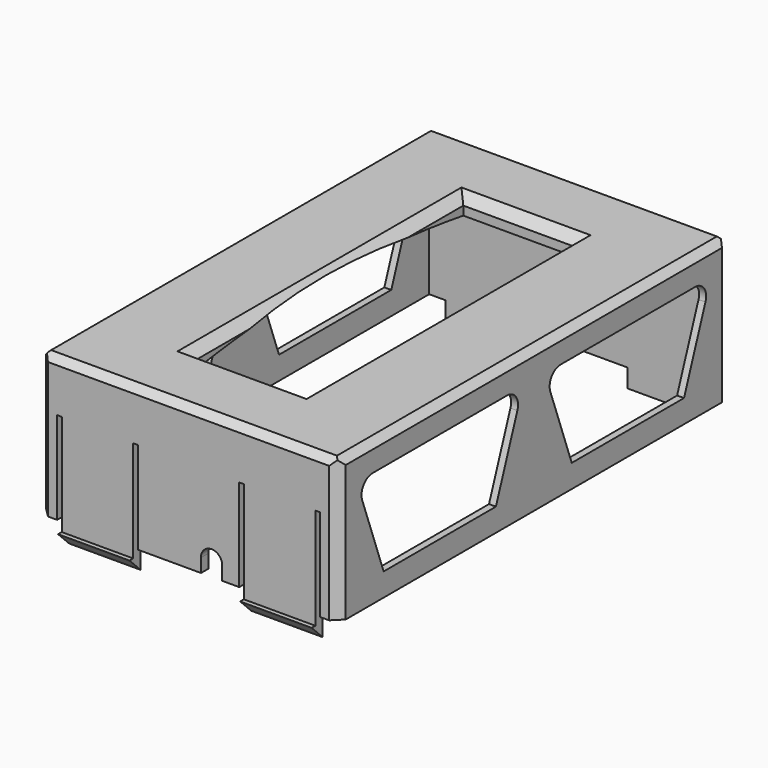
from build123d import *

# Parameters (mm, degrees)
F0_W         = 65
F0_H         = 106
F1_DEPTH     = 31
F3_DEPTH     = 31
F4_W         = 24
F4_H         = 73
F5_DEPTH     = 58
F6_SIZE      = 1.5
F7_T1_DEPTH  = 24
F7_T3_DEPTH  = 73
F7_T9_DEPTH  = 78.1433659759
F7_T13_DEPTH = 29.1433659759
F7_T20_DEPTH = 78.1433659759
F7_T24_DEPTH = 29.1433659759
F7_T31_DEPTH = 29.1433659759
F7_T35_DEPTH = 78.1433659759
F7_T42_DEPTH = 78.1433659759
F7_T46_DEPTH = 29.1433659759
F8_SIZE      = 2
F10_START    = 12
F10_DEPTH    = 15.5
F11_W        = 1
F11_H        = 20
F12_DEPTH    = 2
F14_DEPTH    = 2
F15_R        = 3
F17_DEPTH    = 32.5


# Not quite as in the source:
# - a fillet or chamfer that OpenCascade refuses, or shapes differently, is made with other operations: its cross-section is extruded or revolved along the edge and cut away or added
# - a pattern or mirror of a feature is missing from the dataset's text; its kind, count and spacing are read off the source's solid


with BuildPart() as f1:
    # F0 (on Top) → F1 (new body)
    with BuildSketch(Plane.XY):
        Rectangle(F0_W, F0_H)
    extrude(amount=F1_DEPTH)

    # F2 (on Right) → F3 (cut, symmetric)
    with BuildSketch(Plane.YZ):
        with BuildLine():
            Line((-51, 24.2743855192), (-51, 0))
            Line((-51, 0), (51, 0))
            Line((51, 0), (51, 24.2743855192))
            ThreePointArc((51, 24.2743855192), (0, 30), (-51, 24.2743855192))
        make_face()
    extrude(amount=F3_DEPTH, both=True, mode=Mode.SUBTRACT)

    # F4 (on Top) → F5 (cut)
    with BuildSketch(Plane.XY):
        Rectangle(F4_W, F4_H)
    extrude(amount=F5_DEPTH, mode=Mode.SUBTRACT)

    # F6
    f6_edges = [f1.edges().sort_by_distance(p)[0] for p in [
        (0, 53, 31),
        (-32.5, 0, 31),
        (32.5, 0, 31),
        (0, -53, 31),
    ]]
    chamfer(f6_edges, length=F6_SIZE)

    # F7: chamfer of 2 on 4 edges, made by hand

    # F7_s2 → F7_t1 (cut)
    with BuildSketch(Plane.YZ.offset(-12)):
        Polygon((38.5, 31), (36.5, 29), (36.5, 31), align=None)
        Polygon((-38.5, 31), (-36.5, 29), (-36.5, 31), align=None)
    extrude(amount=F7_T1_DEPTH, mode=Mode.SUBTRACT)

    # F7_s4 → F7_t3 (cut)
    with BuildSketch(Plane.XZ.offset(-36.5)):
        Polygon((14, 31), (12, 29), (12, 31), align=None)
        Polygon((-14, 31), (-12, 29), (-12, 31), align=None)
    extrude(amount=F7_T3_DEPTH, mode=Mode.SUBTRACT)


with BuildPart() as f7_tool7:
    # F7_s8 → F7_t9 (new body)
    with BuildSketch(Plane.XZ.offset(36.5)):
        Polygon((-14, 31), (-12, 29), (-12, 31), align=None)
    extrude(amount=-F7_T9_DEPTH)

    split(bisect_by=Plane.XZ.offset(-36.5), keep=Keep.BOTTOM)


with BuildPart() as f7_tool11:
    # F7_s12 → F7_t13 (new body)
    with BuildSketch(Plane.YZ.offset(-17.1433659759)):
        Polygon((38.5, 31), (36.5, 29), (36.5, 31), align=None)
    extrude(amount=F7_T13_DEPTH)

    split(bisect_by=Plane.YZ.offset(-12), keep=Keep.BOTTOM)


with BuildPart() as f7_tool7_1:
    add(f7_tool7.part)

    # F7_t15: intersect F7_tool11
    add(f7_tool11.part, mode=Mode.INTERSECT)


with BuildPart() as f1_1:
    add(f1.part)

    # F7_t5: cut F7_tool7
    add(f7_tool7_1.part, mode=Mode.SUBTRACT)


with BuildPart() as f7_tool18:
    # F7_s19 → F7_t20 (new body)
    with BuildSketch(Plane.XZ.offset(-41.6433659759)):
        Polygon((14, 31), (12, 29), (12, 31), align=None)
    extrude(amount=F7_T20_DEPTH)

    split(bisect_by=Plane.XZ.offset(-36.5), keep=Keep.BOTTOM)


with BuildPart() as f7_tool22:
    # F7_s23 → F7_t24 (new body)
    with BuildSketch(Plane.YZ.offset(-12)):
        Polygon((38.5, 31), (36.5, 29), (36.5, 31), align=None)
    extrude(amount=F7_T24_DEPTH)

    split(bisect_by=Plane.YZ.offset(12), keep=Keep.TOP)


with BuildPart() as f7_tool18_1:
    add(f7_tool18.part)

    # F7_t26: intersect F7_tool22
    add(f7_tool22.part, mode=Mode.INTERSECT)


with BuildPart() as f1_2:
    add(f1_1.part)

    # F7_t16: cut F7_tool18
    add(f7_tool18_1.part, mode=Mode.SUBTRACT)


with BuildPart() as f7_tool29:
    # F7_s30 → F7_t31 (new body)
    with BuildSketch(Plane.YZ.offset(17.1433659759)):
        Polygon((-38.5, 31), (-36.5, 29), (-36.5, 31), align=None)
    extrude(amount=-F7_T31_DEPTH)

    split(bisect_by=Plane.YZ.offset(12), keep=Keep.TOP)


with BuildPart() as f7_tool33:
    # F7_s34 → F7_t35 (new body)
    with BuildSketch(Plane.XZ.offset(-36.5)):
        Polygon((14, 31), (12, 29), (12, 31), align=None)
    extrude(amount=F7_T35_DEPTH)

    split(bisect_by=Plane.XZ.offset(36.5), keep=Keep.TOP)


with BuildPart() as f7_tool29_1:
    add(f7_tool29.part)

    # F7_t37: intersect F7_tool33
    add(f7_tool33.part, mode=Mode.INTERSECT)


with BuildPart() as f1_3:
    add(f1_2.part)

    # F7_t27: cut F7_tool29
    add(f7_tool29_1.part, mode=Mode.SUBTRACT)


with BuildPart() as f7_tool40:
    # F7_s41 → F7_t42 (new body)
    with BuildSketch(Plane.XZ.offset(41.6433659759)):
        Polygon((-14, 31), (-12, 29), (-12, 31), align=None)
    extrude(amount=-F7_T42_DEPTH)

    split(bisect_by=Plane.XZ.offset(36.5), keep=Keep.TOP)


with BuildPart() as f7_tool44:
    # F7_s45 → F7_t46 (new body)
    with BuildSketch(Plane.YZ.offset(12)):
        Polygon((-38.5, 31), (-36.5, 29), (-36.5, 31), align=None)
    extrude(amount=-F7_T46_DEPTH)

    split(bisect_by=Plane.YZ.offset(-12), keep=Keep.BOTTOM)


with BuildPart() as f7_tool40_1:
    add(f7_tool40.part)

    # F7_t48: intersect F7_tool44
    add(f7_tool44.part, mode=Mode.INTERSECT)


with BuildPart() as f1_4:
    add(f1_3.part)

    # F7_t38: cut F7_tool40
    add(f7_tool40_1.part, mode=Mode.SUBTRACT)

    # F8
    f8_edges = [f1_4.edges().sort_by_distance(p)[0] for p in [
        (-32.5, 53, 14.75),
        (-32.5, -53, 14.75),
        (32.5, -53, 14.75),
        (32.5, 53, 14.75),
    ]]
    chamfer(f8_edges, length=F8_SIZE)

    # F9 (on Right) → F10 (join)
    with BuildSketch(Plane.YZ.offset(F10_START)):
        Polygon((53, 0), (51, 0), (51, -4), (54, -4), (54, -2), (53, -2), align=None)
        Polygon((-51, -5), (-51, 0), (-53, 0), (-53, -2), (-54, -2), align=None)
    f10 = extrude(amount=F10_DEPTH)

    # F10_copies: F10 across plane
    add(f10.mirror(Plane(origin=(0, 0, 0), x_dir=(0, 0, -1), z_dir=(-1, 0, 0))))

    # F11 (on face) → F12 (cut)
    with BuildSketch(Plane.XZ.offset(53)):
        with Locations((28, 10)):
            Rectangle(F11_W, F11_H)
        with Locations((11.5, 10)):
            Rectangle(F11_W, F11_H)
    f12 = extrude(amount=-F12_DEPTH, mode=Mode.SUBTRACT)

    # F12_copies: F12 across plane
    add(f12.mirror(Plane(origin=(0, 0, 0), x_dir=(0, 0, -1), z_dir=(-1, 0, 0))), mode=Mode.SUBTRACT)

    # F13 (on face) → F14 (cut)
    with BuildSketch(Plane.XZ.offset(53)):
        with BuildLine():
            Line((7.299347323, 0), (7.299347323, 2.9452105118))
            ThreePointArc((7.299347323, 2.9452105118), (4.9972996363, 5.2999984148), (2.7007876694, 2.9398114717))
            Line((2.7007876694, 2.9398114717), (2.7007876694, 0))
            Line((2.7007876694, 0), (7.299347323, 0))
        make_face()
    extrude(amount=-F14_DEPTH, mode=Mode.SUBTRACT)

    # F15
    f15_edges = [f1_4.edges().sort_by_distance(p)[0] for p in [
        (0, -51, 24.274386),
        (-31, 0, 30),
        (31, 0, 30),
        (0, 51, 24.274386),
    ]]
    fillet(f15_edges, radius=F15_R)

    # F16 (on Right) → F17 (cut, symmetric)
    with BuildSketch(Plane.YZ):
        with BuildLine():
            Line((40.7205953147, 5), (46.5346338421, 20.97393957))
            ThreePointArc((46.5346338421, 20.97393957), (46.1730121126, 23.7207293091), (43.7155559798, 25))
            Line((43.7155559798, 25), (7.2844440202, 25))
            ThreePointArc((7.2844440202, 25), (4.8269878874, 23.7207293091), (4.4653661579, 20.97393957))
            Line((4.4653661579, 20.97393957), (10.2794046853, 5))
            Line((10.2794046853, 5), (40.7205953147, 5))
        make_face()
        with BuildLine():
            Line((-40.7205953147, 5), (-10.2794046853, 5))
            Line((-10.2794046853, 5), (-4.4653661579, 20.97393957))
            ThreePointArc((-4.4653661579, 20.97393957), (-4.8269878874, 23.7207293091), (-7.2844440202, 25))
            Line((-7.2844440202, 25), (-43.7155559798, 25))
            ThreePointArc((-43.7155559798, 25), (-46.1730121126, 23.7207293091), (-46.5346338421, 20.97393957))
            Line((-46.5346338421, 20.97393957), (-40.7205953147, 5))
        make_face()
    extrude(amount=F17_DEPTH, both=True, mode=Mode.SUBTRACT)


solid = f1_4.part
